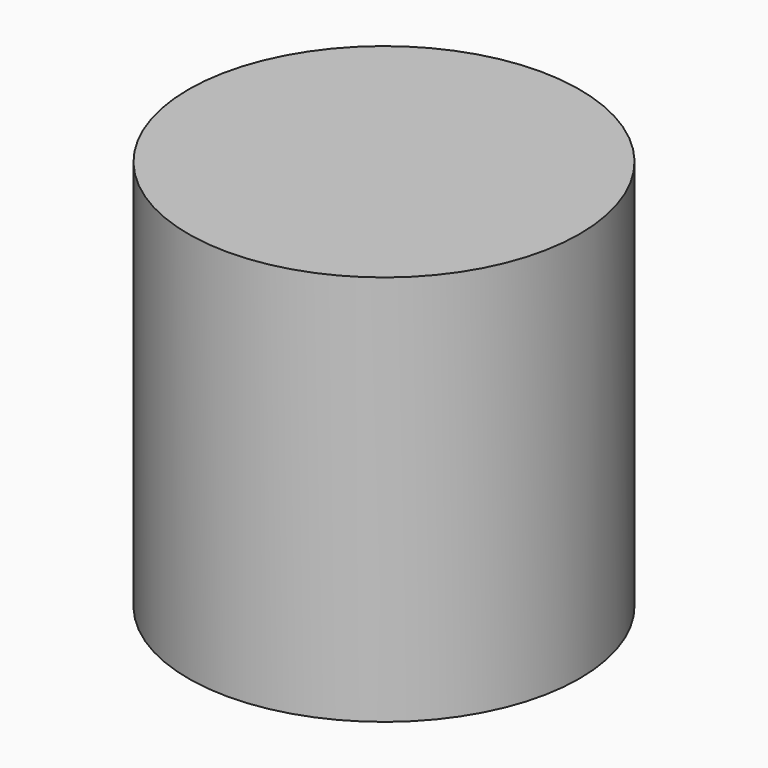
from build123d import *

# Parameters (mm, degrees)
F0_R     = 63.5
F1_DEPTH = 127


# Not quite as in the source:
# - the program builds the solid bodies; features that only make, move or delete a surface that nothing else refers to are left out


with BuildPart() as f1:
    # F0 (on Top) → F1 (new body)
    with BuildSketch(Plane.XY):
        Circle(F0_R)
    extrude(amount=F1_DEPTH)


solid = f1.part
